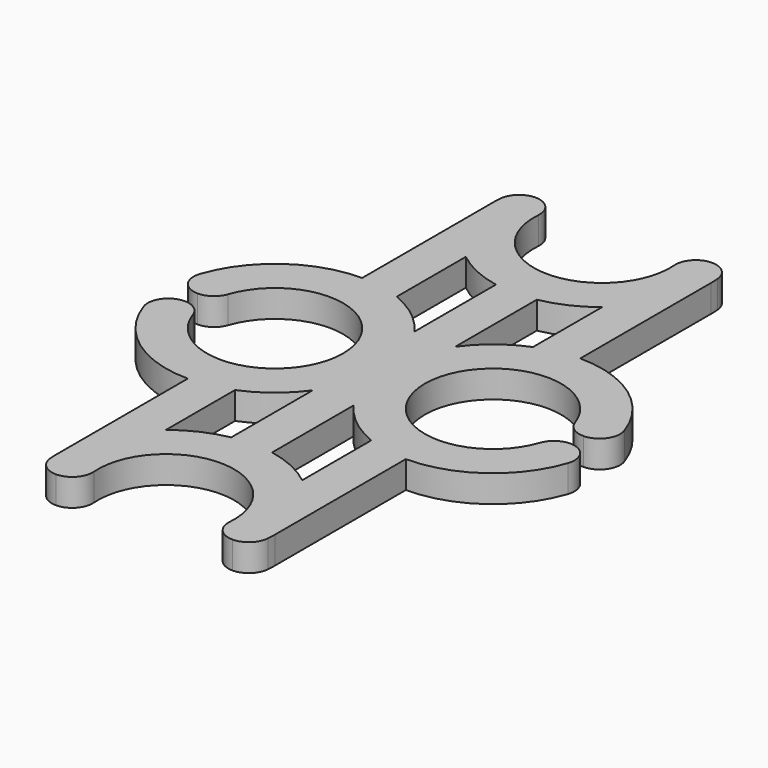
from build123d import *

# Parameters (mm, degrees)
F1_DEPTH = 2.54
F2_R     = 6.35
F3_DEPTH = 25.4
F5_DEPTH = 2.54
F6_W     = 18.9905706793
F6_H     = 1.524
F7_DEPTH = 25.4
F8_R     = 1.90499


# Not quite as in the source:
# - a fillet or chamfer is up to 0.001 mm smaller than in the source, because OpenCascade refuses the exact size


with BuildPart() as f1:
    # F0 (on Top) → F1 (new body)
    with BuildSketch(Plane.XY):
        with BuildLine():
            Line((9.8373776994, 27.94), (-9.8373776994, 27.94))
            ThreePointArc((-9.8373776994, 27.94), (-8.5823807234, 19.962322084), (-1.905, 15.4201916351))
            Line((-1.905, 15.4201916351), (-1.905, 25.4))
            Line((-1.905, 25.4), (1.905, 25.4))
            Line((1.905, 25.4), (1.905, 15.4201916351))
            ThreePointArc((1.905, 15.4201916351), (8.5823807234, 19.962322084), (9.8373776994, 27.94))
        make_face()
        with BuildLine():
            Line((-1.905, 25.4), (-1.905, 15.4201916351))
            ThreePointArc((-1.905, 15.4201916351), (0, 15.24), (1.905, 15.4201916351))
            Line((1.905, 15.4201916351), (1.905, 25.4))
            Line((1.905, 25.4), (-1.905, 25.4))
        make_face()
        with BuildLine():
            ThreePointArc((1.905, 15.4201916351), (0, 15.24), (-1.905, 15.4201916351))
            Line((-1.905, 15.4201916351), (-1.905, 5.9228856987))
            ThreePointArc((-1.905, 5.9228856987), (-0.4879681556, 3.1108519733), (0, 0))
            ThreePointArc((0, 0), (0.4879681556, 3.1108519733), (1.905, 5.9228856987))
            Line((1.905, 5.9228856987), (1.905, 15.4201916351))
        make_face()
        with BuildLine():
            ThreePointArc((0, 0), (-0.4879681556, 3.1108519733), (-1.905, 5.9228856987))
            Line((-1.905, 5.9228856987), (-1.905, -5.9228856987))
            ThreePointArc((-1.905, -5.9228856987), (-0.4879681556, -3.1108519733), (0, 0))
        make_face()
        with BuildLine():
            Line((-1.905, -5.9228856987), (-1.905, 5.9228856987))
            ThreePointArc((-1.905, 5.9228856987), (-20.32, 0), (-1.905, -5.9228856987))
        make_face()
        with BuildLine():
            ThreePointArc((20.32, 0), (13.2708519733, 9.6720318444), (1.905, 5.9228856987))
            Line((1.905, 5.9228856987), (1.905, -5.9228856987))
            ThreePointArc((1.905, -5.9228856987), (13.2708519733, -9.6720318444), (20.32, 0))
        make_face()
        with BuildLine():
            Line((1.905, -5.9228856987), (1.905, 5.9228856987))
            ThreePointArc((1.905, 5.9228856987), (0.4879681556, 3.1108519733), (0, 0))
            ThreePointArc((0, 0), (0.4879681556, -3.1108519733), (1.905, -5.9228856987))
        make_face()
        with BuildLine():
            ThreePointArc((0, 0), (-0.4879681556, -3.1108519733), (-1.905, -5.9228856987))
            Line((-1.905, -5.9228856987), (-1.905, -15.4201916351))
            ThreePointArc((-1.905, -15.4201916351), (0, -15.24), (1.905, -15.4201916351))
            Line((1.905, -15.4201916351), (1.905, -5.9228856987))
            ThreePointArc((1.905, -5.9228856987), (0.4879681556, -3.1108519733), (0, 0))
        make_face()
        with BuildLine():
            Line((-1.905, -25.4), (-1.905, -15.4201916351))
            ThreePointArc((-1.905, -15.4201916351), (-8.5823807234, -19.962322084), (-9.8373776994, -27.94))
            Line((-9.8373776994, -27.94), (9.8373776994, -27.94))
            ThreePointArc((9.8373776994, -27.94), (8.5823807234, -19.962322084), (1.905, -15.4201916351))
            Line((1.905, -15.4201916351), (1.905, -25.4))
            Line((1.905, -25.4), (-1.905, -25.4))
        make_face()
        with BuildLine():
            ThreePointArc((1.905, -15.4201916351), (0, -15.24), (-1.905, -15.4201916351))
            Line((-1.905, -15.4201916351), (-1.905, -25.4))
            Line((-1.905, -25.4), (1.905, -25.4))
            Line((1.905, -25.4), (1.905, -15.4201916351))
        make_face()
    extrude(amount=F1_DEPTH)

    # F2 (on face) → F3 (cut)
    with BuildSketch(Plane.XY.offset(2.54)):
        with Locations((0, 25.4)):
            Circle(F2_R)
        with Locations((10.16, 0)):
            Circle(F2_R)
        with Locations((-10.16, 0)):
            Circle(F2_R)
        with Locations((0, -25.4)):
            Circle(F2_R)
    extrude(amount=-F3_DEPTH, mode=Mode.SUBTRACT)

    # F4 (on face) → F5 (join, through all)
    with BuildSketch(Plane.XY.offset(2.54)):
        with BuildLine():
            ThreePointArc((6.35, -17.468852542), (9.1581002397, -21.0005909488), (10.16, -25.4))
            Line((10.16, -25.4), (10.16, -10.16))
            ThreePointArc((10.16, -10.16), (8.2192646134, -9.9729206434), (6.35, -9.4185720786))
            Line((6.35, -9.4185720786), (6.35, -17.468852542))
        make_face()
        with BuildLine():
            ThreePointArc((-10.16, -25.4), (-9.1581002397, -21.0005909488), (-6.35, -17.468852542))
            Line((-6.35, -17.468852542), (-6.35, -9.4185720786))
            ThreePointArc((-6.35, -9.4185720786), (-8.2192646134, -9.9729206434), (-10.16, -10.16))
            Line((-10.16, -10.16), (-10.16, -25.4))
        make_face()
        with BuildLine():
            Line((10.16, 10.16), (10.16, 25.4))
            ThreePointArc((10.16, 25.4), (9.1581002397, 21.0005909488), (6.35, 17.468852542))
            Line((6.35, 17.468852542), (6.35, 9.4185720786))
            ThreePointArc((6.35, 9.4185720786), (8.2192646134, 9.9729206434), (10.16, 10.16))
        make_face()
        with BuildLine():
            ThreePointArc((-6.35, 17.468852542), (-9.1581002397, 21.0005909488), (-10.16, 25.4))
            Line((-10.16, 25.4), (-10.16, 10.16))
            ThreePointArc((-10.16, 10.16), (-8.2192646134, 9.9729206434), (-6.35, 9.4185720786))
            Line((-6.35, 9.4185720786), (-6.35, 17.468852542))
        make_face()
    extrude(amount=-F5_DEPTH)

    # F6 (on face) → F7 (cut)
    with BuildSketch(Plane.XY.offset(2.54)):
        with Locations((19.6552853397, 0)):
            Rectangle(F6_W, F6_H)
        with Locations((-19.6552853397, 0)):
            Rectangle(F6_W, F6_H)
    extrude(amount=-F7_DEPTH, mode=Mode.SUBTRACT)

    # F8 (radius 1.905 in the source; OpenCascade refuses exactly that, so slightly less here)
    f8_edges = [f1.edges().sort_by_distance(p)[0] for p in [
        (20.291385, -0.762, 1.27),
        (20.291385, 0.762, 1.27),
        (16.464114, -0.762, 1.27),
        (16.464114, 0.762, 1.27),
        (5.819871, -27.94, 1.27),
        (-5.819871, -27.94, 1.27),
        (9.837378, -27.94, 1.27),
        (-20.291385, 0.762, 1.27),
        (-20.291385, -0.762, 1.27),
        (-16.464114, -0.762, 1.27),
        (-16.464114, 0.762, 1.27),
        (-9.837378, 27.94, 1.27),
        (5.819871, 27.94, 1.27),
        (-5.819871, 27.94, 1.27),
        (9.837378, 27.94, 1.27),
        (-9.837378, -27.94, 1.27),
    ]]
    fillet(f8_edges, radius=F8_R)


solid = f1.part
